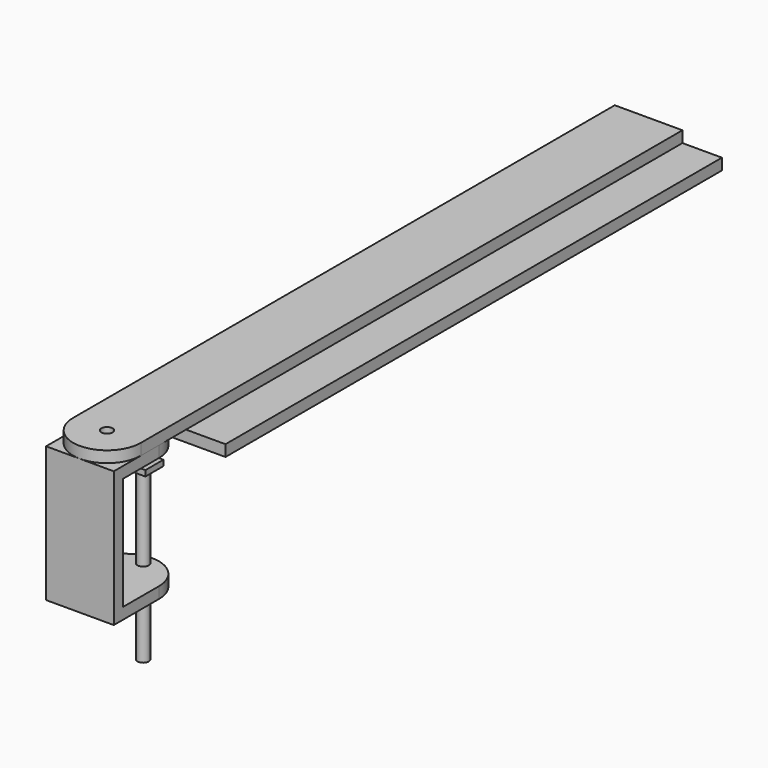
from build123d import *

# Parameters (mm, degrees)
F1_W           = 60
F1_H           = 550
F2_DEPTH       = 20
F1_W_2         = 35
F3_DEPTH       = 10
F1_R           = 5
F4_DEPTH       = 20
F5_DEPTH       = 10
F6_W           = 60
F6_H           = 10
F7_DEPTH       = 10
F8_DEPTH       = 100
F9_R           = 5
F9_W           = 60
F9_H           = 10
F10_DEPTH      = 10
F11_R          = 5
F12_DEPTH      = 75
F12_DEPTH_BACK = 75
F13_W          = 20.000001848
F13_H          = 20.000001848
F13_R          = 5
F14_DEPTH      = 5


with BuildPart() as f2:
    # F1 (on Top) → F2 (new body)
    with BuildSketch(Plane.XY):
        with Locations((-30, 275)):
            Rectangle(F1_W, F1_H)
    extrude(amount=F2_DEPTH)

    # F1 (on Top) → F3 (join)
    with BuildSketch(Plane.XY):
        with Locations((17.5, 275)):
            Rectangle(F1_W_2, F1_H)
    extrude(amount=F3_DEPTH)

    # F1 (on Top) → F4 (join)
    with BuildSketch(Plane.XY):
        with BuildLine():
            Line((0, -50), (0, 0))
            Line((0, 0), (-60, 0))
            Line((-60, 0), (-60, -50))
            ThreePointArc((-60, -50), (-30, -80), (0, -50))
        make_face()
        with Locations((-30, -50)):
            Circle(F1_R, mode=Mode.SUBTRACT)
    extrude(amount=F4_DEPTH)

    # F1 (on Top) → F5 (cut)
    with BuildSketch(Plane.XY):
        with BuildLine():
            Line((0, -50), (0, 0))
            Line((0, 0), (-60, 0))
            Line((-60, 0), (-60, -50))
            ThreePointArc((-60, -50), (-30, -80), (0, -50))
        make_face()
        with Locations((-30, -50)):
            Circle(F1_R, mode=Mode.SUBTRACT)
    extrude(amount=F5_DEPTH, mode=Mode.SUBTRACT)


with BuildPart() as f7:
    # F6 (on face) → F7 (new body)
    with BuildSketch(Plane(origin=(0, 0, 0), x_dir=(1, 0, 0), z_dir=(0, 0, -1))):
        with Locations((-30, 75)):
            Rectangle(F6_W, F6_H)
        with BuildLine():
            Line((-60, 70), (-60, 30))
            ThreePointArc((-60, 30), (-51.2132034519, 8.7867965807), (-30.0000000462, 0))
            ThreePointArc((-30.0000000462, 0), (-8.7867965807, 8.7867965481), (0, 30))
            Line((0, 30), (0, 70))
            Line((0, 70), (-60, 70))
        make_face()
    extrude(amount=-F7_DEPTH)

    # F6 (on face) → F8 (join)
    with BuildSketch(Plane(origin=(0, 0, 0), x_dir=(1, 0, 0), z_dir=(0, 0, -1))):
        with Locations((-30, 75)):
            Rectangle(F6_W, F6_H)
    extrude(amount=F8_DEPTH)

    # F9 (on face) → F10 (join)
    with BuildSketch(Plane(origin=(0, 0, -100), x_dir=(1, 0, 0), z_dir=(0, 0, -1))):
        with BuildLine():
            Line((0, 70), (-60, 70))
            Line((-60, 70), (-60, 30))
            ThreePointArc((-60, 30), (-51.2132034356, 8.7867965644), (-30, 0))
            ThreePointArc((-30, 0), (-8.7867965644, 8.7867965644), (0, 30))
            Line((0, 30), (0, 70))
        make_face()
        with Locations((-30, 10)):
            Circle(F9_R, mode=Mode.SUBTRACT)
        with Locations((-30, 75)):
            Rectangle(F9_W, F9_H)
    extrude(amount=F10_DEPTH)


with BuildPart() as f12:
    # F11 (on face) → F12 (new body, two sides)
    with BuildSketch(Plane.XY.offset(-100)) as f12_sk:
        with Locations((-29.9999999688, -10)):
            Circle(F11_R)
    extrude(amount=F12_DEPTH)
    extrude(f12_sk.sketch, amount=-F12_DEPTH_BACK)

    # F13 (on face) → F14 (join)
    with BuildSketch(Plane.XY.offset(-25)):
        with Locations((-30, -10.000000924)):
            Rectangle(F13_W, F13_H)
        with Locations((-29.9999999688, -10)):
            Circle(F13_R, mode=Mode.SUBTRACT)
        with Locations((-30, -10.000000924)):
            Rectangle(F13_W, F13_H)
    extrude(amount=F14_DEPTH)


solid = Compound([f2.part, f7.part, f12.part])
